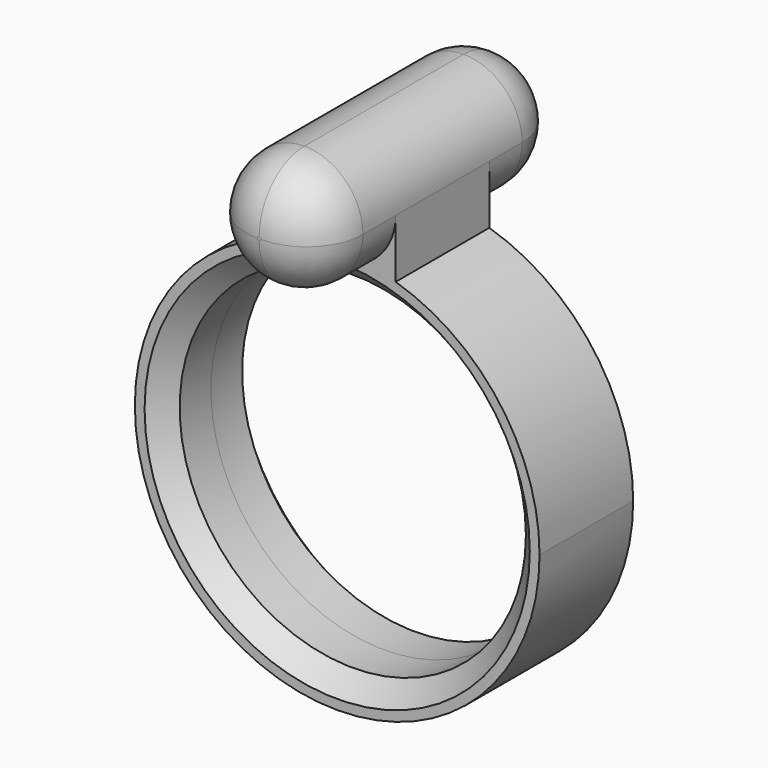
from build123d import *

# Parameters (mm, degrees)
F0_R          = 8.875
F1_DEPTH      = 3
F1_DEPTH_BACK = 3
F2_SIZE       = 1
F3_DEPTH      = 8
F3_DEPTH_BACK = 8
F4_R          = 2.99999
F5_R          = 2.9


# Not quite as in the source:
# - a fillet or chamfer is up to 0.001 mm smaller than in the source, because OpenCascade refuses the exact size
# - a feature names something its author has since deleted; it is built from what else it names


with BuildPart() as f1:
    # F0 (on Front) → F1 (new body, two sides)
    with BuildSketch(Plane.XZ) as f1_sk:
        with BuildLine():
            ThreePointArc((-3, 9.931798679), (-6.1852900094, -8.3296345958), (10.375, 0))
            ThreePointArc((10.375, 0), (8.3296345958, 6.1852900094), (3, 9.931798679))
            Line((3, 9.931798679), (-3, 9.931798679))
        make_face()
        Circle(F0_R, mode=Mode.SUBTRACT)
    extrude(amount=F1_DEPTH)
    extrude(f1_sk.sketch, amount=-F1_DEPTH_BACK)

    # F2
    f2_edges = [f1.edges().sort_by_distance(p)[0] for p in [
        (-8.875, -3, 0),
        (-8.875, 3, 0),
    ]]
    chamfer(f2_edges, length=F2_SIZE)

    # F0 (on Front) → F3 (join, two sides)
    with BuildSketch(Plane.XZ) as f3_sk:
        with BuildLine():
            ThreePointArc((-3, 9.931798679), (0, 10.375), (3, 9.931798679))
            Line((3, 9.931798679), (3, 15.931798679))
            Line((3, 15.931798679), (-3, 15.931798679))
            Line((-3, 15.931798679), (-3, 9.931798679))
        make_face()
        with BuildLine():
            Line((-3, 9.931798679), (3, 9.931798679))
            ThreePointArc((3, 9.931798679), (0, 10.375), (-3, 9.931798679))
        make_face()
    extrude(amount=F3_DEPTH)
    extrude(f3_sk.sketch, amount=-F3_DEPTH_BACK)

    # F4 (radius 3 in the source; OpenCascade refuses exactly that, so slightly less here)
    f4_edges = [f1.edges().sort_by_distance(p)[0] for p in [
        (-3, 0, 15.931799),
        (3, 0, 15.931799),
        (3, -5.5, 9.931799),
        (3, 5.5, 9.931799),
        (-3, -5.5, 9.931799),
        (-3, 5.5, 9.931799),
    ]]
    fillet(f4_edges, radius=F4_R)

    # F5
    f5_edges = [f1.edges().sort_by_distance(p)[0] for p in [
        (2.121323, -8, 15.053122),
        (2.121323, 8, 15.053122),
        (3, -8, 12.931799),
        (3, 8, 12.931799),
        (2.121323, -8, 10.810475),
        (0, -8, 9.931799),
        (0, -8, 15.931799),
        (-2.121323, -8, 10.810475),
        (-2.121323, -8, 15.053122),
        (-3, -8, 12.931799),
        (2.121323, 8, 10.810475),
        (0, 8, 9.931799),
        (0, 8, 15.931799),
        (-2.121323, 8, 10.810475),
        (-2.121323, 8, 15.053122),
        (-3, 8, 12.931799),
    ]]
    fillet(f5_edges, radius=F5_R)


solid = f1.part
